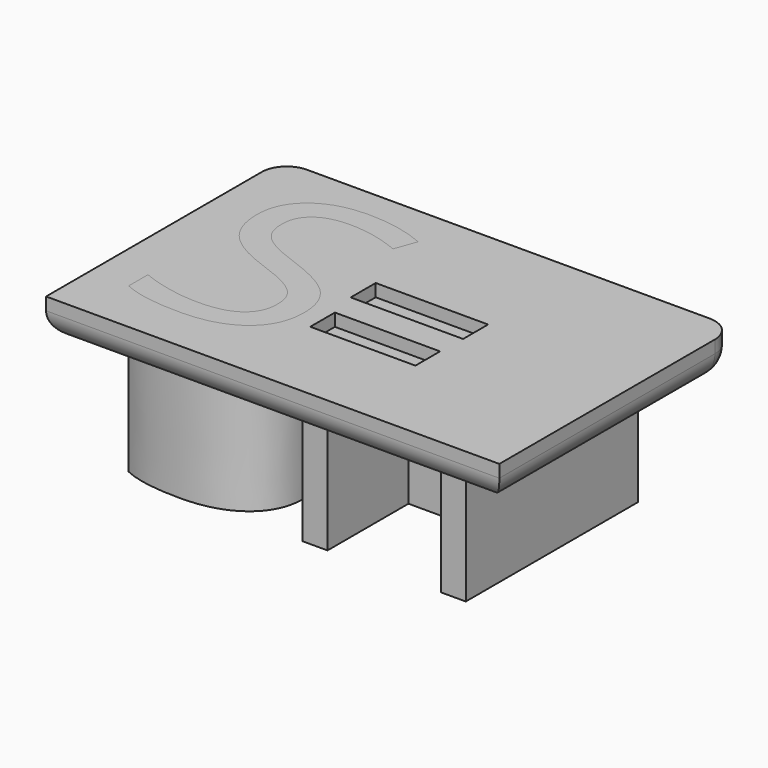
from build123d import *

# Parameters (mm, degrees)
F0_TEXT_SIZE = 60.7700934579
F1_DEPTH     = 25.4
F2_W         = 91.43999964
F2_H         = 59.4360008836
F3_DEPTH     = 7.62
F4_DEPTH     = 7.62
F5_R         = 5.08
F6_W         = 22.6771214511
F6_H         = 6.3093602657
F7_DEPTH     = 2.54
F8_R         = 5.08
F9_W         = 21.2140814401
F9_H         = 6.2179202214
F10_DEPTH    = 2.54


# Not quite as in the source:
# - Text() gives the source's letters only with a copy of the font that has no kerning and outlines rounded to 1/6400 em; it was checked with that copy


with BuildPart() as f1:
    # F0 (on Top) → F1 (new body)
    with BuildSketch(Plane.XY):
        with Locations((-30.1712424612, -20.1526775738)):
            Text('SH', F0_TEXT_SIZE, font='Open Sans', text_align=(TextAlign.LEFT, TextAlign.BOTTOM))
    extrude(amount=F1_DEPTH)

    # F2 (on face) → F3 (join)
    with BuildSketch(Plane.XY.offset(25.4)):
        with Locations((10.7899196446, 0)):
            Rectangle(F2_W, F2_H)
        with BuildLine():
            add(Edge.make_bspline(
                [(-27.0282891902, -18.7568644897), (-22.8693359191, -20.7508831813), (-8.0376349846, -20.7508831813), (0.2707762304, -14.3320420598), (0.2707762304, -4.1625467327), (-4.8567004051, 1.4207056037), (-11.683840592, 3.851509342)],
                knots=[0, 0, 0, 1, 1.9236453202, 2.8472906404, 3.5641496949, 4.2810087494, 4.2810087494, 4.2810087494], degree=2))
            Line((-27.0282891902, -18.7568644897), (-27.0282891902, -13.8952570131))
            add(Edge.make_bspline(
                [(-15.2161022743, 0.0248925196), (-10.8862331154, -1.513350471), (-6.6418219005, -3.9536495365), (-4.8282144238, -6.8307336486), (-4.8282144238, -12.499443929), (-9.9367004051, -16.3260607514), (-18.0647004051, -16.3260607514), (-24.3506069472, -15.0157056112), (-27.0282891902, -13.8952570131)],
                knots=[0, 0, 0, 1, 2, 3, 4.5189873418, 6.0379746835, 6.967675034, 7.8973753844, 7.8973753844, 7.8973753844], degree=2))
            add(Edge.make_bspline(
                [(-0.8211863864, 21.4748364448), (-6.2525134892, 23.8486682205), (-18.9287751715, 23.8486682205), (-26.458569564, 17.9140887813), (-26.458569564, 8.1244065383), (-21.2646256388, 2.1898270991), (-15.2161022743, 0.0248925196)],
                knots=[0, 0, 0, 1, 1.9603524229, 2.9207048458, 3.8355860366, 4.7504672273, 4.7504672273, 4.7504672273], degree=2))
            Line((-0.8211863864, 21.4748364448), (-2.3974106855, 17.0879953234))
            add(Edge.make_bspline(
                [(-11.683840592, 3.851509342), (-15.747840592, 5.3042943888), (-19.6978966668, 7.7066121458), (-21.3595789098, 10.593191585), (-21.3595789098, 15.9010794355), (-16.849298536, 19.3383878467), (-7.7717658257, 19.3383878467), (-2.3974106855, 17.0879953234)],
                knots=[0, 0, 0, 1, 2, 3, 4.358649789, 5.7172995781, 7.4365388846, 7.4365388846, 7.4365388846], degree=2))
        make_face(mode=Mode.SUBTRACT)
    extrude(amount=F3_DEPTH)


with BuildPart() as f4:
    # F4 (new): a face of the model
    f4_faces = [f1.part.faces().sort_by_distance(p)[0] for p in [
        (-13.4059357915, 1.2625830345, 25.4),
    ]]
    extrude(f4_faces, amount=F4_DEPTH)


with BuildPart() as f1_1:
    add(f1.part)

    # F5
    f5_edges = [f1_1.edges().sort_by_distance(p)[0] for p in [
        (-34.93008, 0, 25.4),
        (10.78992, -29.718, 25.4),
        (56.509919, 0, 25.4),
    ]]
    fillet(f5_edges, radius=F5_R)

    # F6 (on face) → F7 (cut)
    with BuildSketch(Plane.XY.offset(33.02)):
        with Locations((14.0817604261, 3.1546801329)):
            Rectangle(F6_W, F6_H)
    extrude(amount=-F7_DEPTH, mode=Mode.SUBTRACT)

    # F8
    f8_edges = [f1_1.edges().sort_by_distance(p)[0] for p in [
        (10.78992, 29.718, 25.4),
    ]]
    fillet(f8_edges, radius=F8_R)

    # F9 (on face) → F10 (cut)
    with BuildSketch(Plane.XY.offset(33.02)):
        with Locations((14.6304003429, -8.6868000217)):
            Rectangle(F9_W, F9_H)
    extrude(amount=-F10_DEPTH, mode=Mode.SUBTRACT)


solid = Compound([f4.part, f1_1.part])
